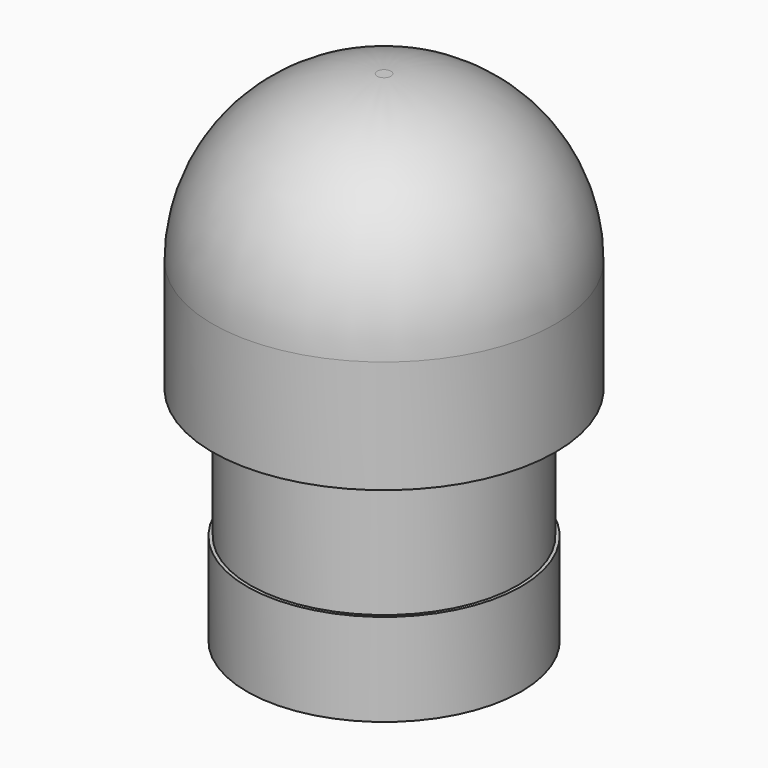
from build123d import *

# Parameters (mm, degrees)
F0_R     = 1.8384679537
F1_DEPTH = 1.778
F2_R     = 2.3552905633
F2_R_2   = 1.8384679537
F3_DEPTH = 3.81
F4_R     = 2.2606
F5_R     = 1.884215831
F5_R_2   = 1.8384679537
F6_DEPTH = 1.27


with BuildPart() as f1:
    # F0 (on Top) → F1 (new body)
    with BuildSketch(Plane.XY):
        Circle(F0_R)
    extrude(amount=F1_DEPTH)


with BuildPart() as f3:
    # F2 (on face) → F3 (new body)
    with BuildSketch(Plane.XY.offset(1.778)):
        Circle(F2_R)
        Circle(F2_R_2, mode=Mode.SUBTRACT)
        Circle(F2_R_2)
    extrude(amount=F3_DEPTH)

    # F4
    f4_edges = [f3.edges().sort_by_distance(p)[0] for p in [
        (-2.355291, 0, 5.588),
    ]]
    fillet(f4_edges, radius=F4_R)


with BuildPart() as f6:
    # F5 (on face) → F6 (new body)
    with BuildSketch(Plane(origin=(0, 0, 0), x_dir=(1, 0, 0), z_dir=(0, 0, -1))):
        Circle(F5_R)
        Circle(F5_R_2, mode=Mode.SUBTRACT)
        Circle(F5_R_2)
    extrude(amount=F6_DEPTH)


solid = Compound([f1.part, f3.part, f6.part])
